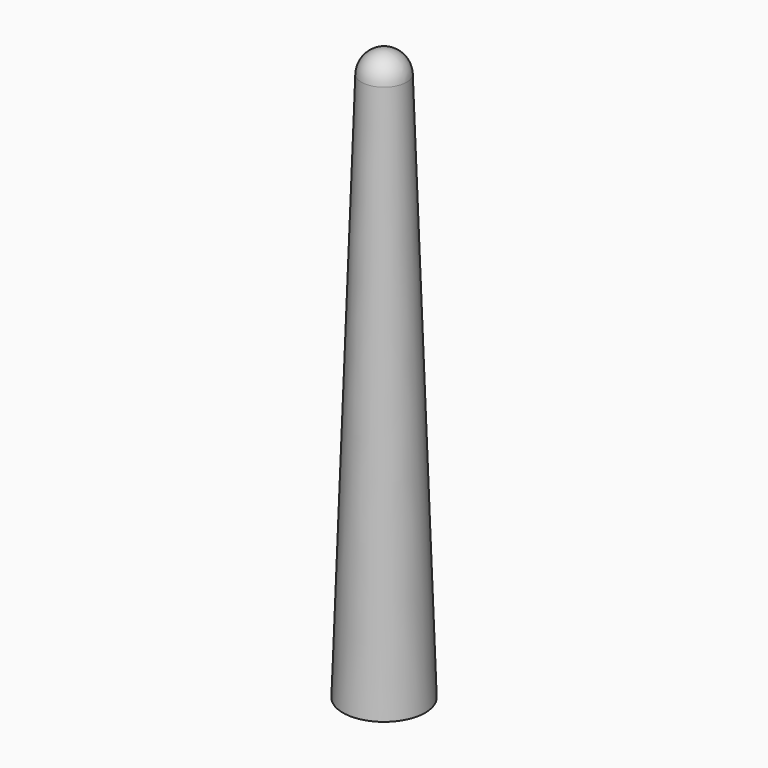
from build123d import *


# Not quite as in the source:
# - a feature of the source that left no trace in its solid (it failed there, or was rolled back) is left out
# - a feature names something its author has since deleted; it is built from what else it names


with BuildPart() as f1:
    # F0 (on Front) → F1 (revolve)
    with BuildSketch(Plane.XZ):
        with BuildLine():
            Line((8.2452101406, -109.7828151841), (4.4973873494, 0.1533200233))
            ThreePointArc((4.4973873494, 0.1533200233), (3.1273039423, 3.2357333098), (0, 4.5))
            Line((0, 4.5), (0, 2.8))
            ThreePointArc((0, 2.8), (1.9458780086, 2.0133451706), (2.7983743507, 0.0953991256))
            Line((2.7983743507, 0.0953991256), (6.4590447751, -107.2842666566))
            Line((6.4590447751, -107.2842666566), (6.4726732216, -107.684034421))
            Line((6.4726732216, -107.684034421), (6.4863016682, -108.0838021854))
            Line((6.4863016682, -108.0838021854), (6.5033471227, -108.5838021854))
            Line((6.5033471227, -108.5838021854), (6.5442225658, -109.7828151841))
            Line((6.5442225658, -109.7828151841), (8.2452101406, -109.7828151841))
        make_face()
        with BuildLine():
            Line((6.4726732216, -107.684034421), (6.4590447751, -107.2842666566))
            ThreePointArc((6.4590447751, -107.2842666566), (6.2505990382, -107.4374019066), (6.1726732216, -107.684034421))
            Line((6.1726732216, -107.684034421), (6.4726732216, -107.684034421))
        make_face()
        with BuildLine():
            ThreePointArc((6.1726732216, -107.684034421), (6.2615032541, -107.9372537095), (6.4863016682, -108.0838021854))
            Line((6.4863016682, -108.0838021854), (6.4726732216, -107.684034421))
            Line((6.4726732216, -107.684034421), (6.1726732216, -107.684034421))
        make_face()
    revolve(axis=Axis((0, 0, -52.7819509467), (0, 0, 1)))


solid = f1.part
